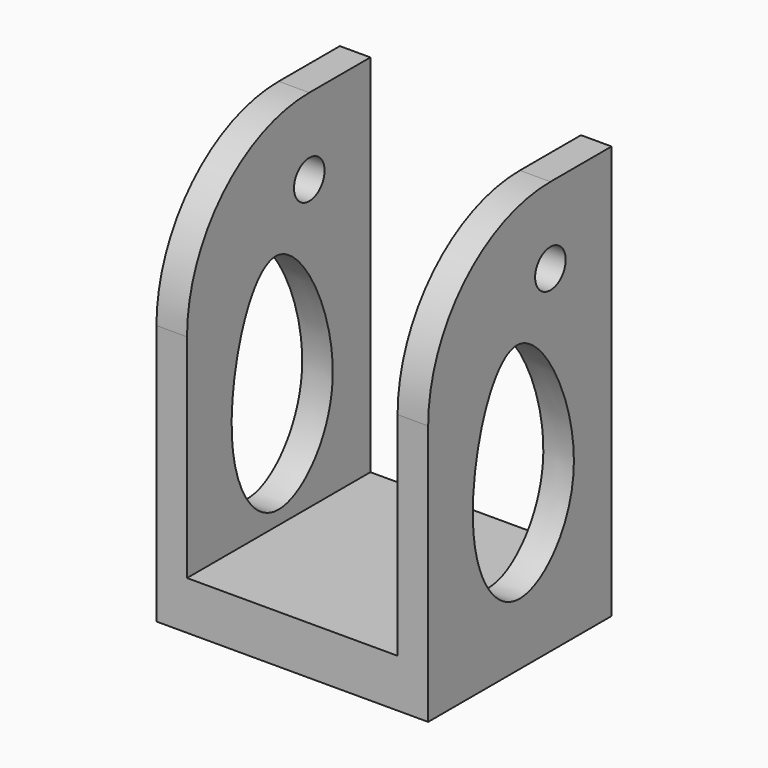
from build123d import *

# Parameters (mm, degrees)
F0_W     = 5.08
F0_H     = 60.6926516568
F1_DEPTH = 38.1
F3_D     = 6.35
F4_DEPTH = 45.161
F5_R     = 25.4


# Not quite as in the source:
# - a feature names something its author has since deleted; it is built from what else it names


with BuildPart() as f1:
    # F0 (on Front) → F1 (new body)
    with BuildSketch(Plane.XZ):
        Polygon((-45.16, 0), (0, 0), (0, 8.0210549811), (-5.08, 8.0210549811), (-40.08, 8.0210549811), (-45.16, 8.0210549811), align=None)
        with Locations((-2.54, 38.3673808095)):
            Rectangle(F0_W, F0_H)
        with Locations((-42.62, 38.3673808095)):
            Rectangle(F0_W, F0_H)
    extrude(amount=F1_DEPTH)

    # F3 (through all)
    with Locations(Plane.YZ):
        with Locations((-12.7, 56.0137066379)):
            Hole(F3_D / 2)

    # F2 (on Right) → F4 (cut, through all)
    with BuildSketch(Plane.YZ):
        with BuildLine():
            add(Edge.make_bspline(
                [(-19.1434975713, 10.3080365807), (-23.9365403388, 10.3492805031), (-32.9940706123, 22.9579895891), (-21.1738830705, 60.90718063), (-1.4242230003, 23.6437509657), (-14.1250016542, 10.2648526438), (-19.1434975713, 10.3080365807)],
                knots=[0, 0, 0, 0, 0.2215384982, 0.4930848573, 0.7680408662, 1, 1, 1, 1], degree=3))
        make_face()
    extrude(amount=-F4_DEPTH, mode=Mode.SUBTRACT)

    # F5
    f5_edges = [f1.edges().sort_by_distance(p)[0] for p in [
        (-2.54, -38.1, 68.713707),
        (-42.62, -38.1, 68.713707),
    ]]
    fillet(f5_edges, radius=F5_R)


solid = f1.part
